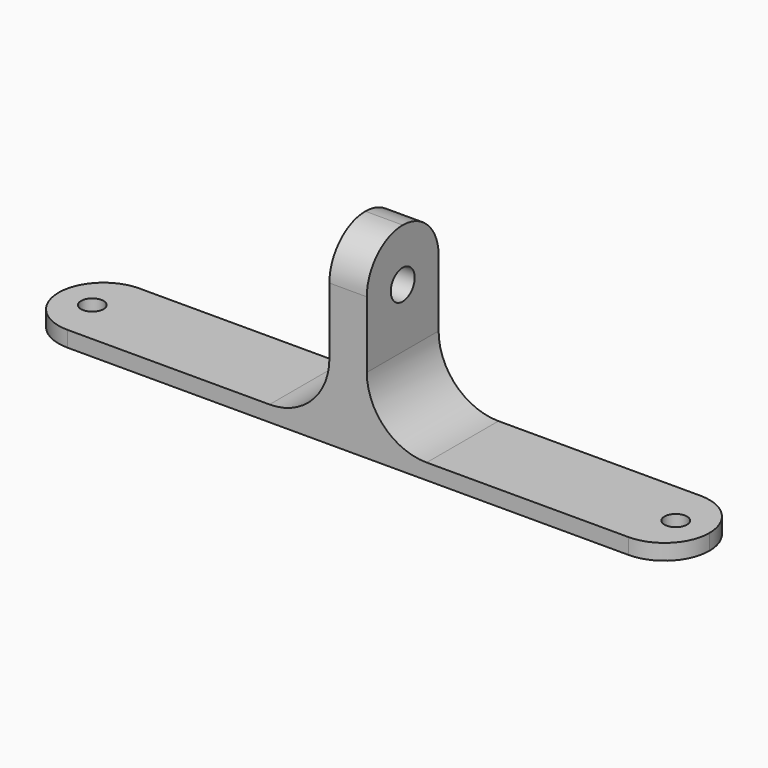
from build123d import *

# Parameters (mm, degrees)
F0_W     = 41
F0_H     = 12
F0_R     = 1.5
F0_W_2   = 5
F1_DEPTH = 2.1
F2_DEPTH = 25
F3_R     = 2
F4_DEPTH = 12.5
F5_R     = 5.99999
F6_R     = 8


# Not quite as in the source:
# - a fillet or chamfer is up to 0.001 mm smaller than in the source, because OpenCascade refuses the exact size


with BuildPart() as f1:
    # F0 (on Top) → F1 (new body)
    with BuildSketch(Plane.XY):
        with Locations((-23, 0)):
            Rectangle(F0_W, F0_H)
        with Locations((-39, 0)):
            Circle(F0_R, mode=Mode.SUBTRACT)
        Rectangle(F0_W_2, F0_H)
        with Locations((23, 0)):
            Rectangle(F0_W, F0_H)
        with Locations((39, 0)):
            Circle(F0_R, mode=Mode.SUBTRACT)
    extrude(amount=F1_DEPTH)

    # F0 (on Top) → F2 (join)
    with BuildSketch(Plane.XY):
        Rectangle(F0_W_2, F0_H)
    extrude(amount=F2_DEPTH)

    # F3 (on Right) → F4 (cut, symmetric)
    with BuildSketch(Plane.YZ):
        with Locations((0, 18)):
            Circle(F3_R)
    extrude(amount=F4_DEPTH, both=True, mode=Mode.SUBTRACT)

    # F5 (radius 6 in the source; OpenCascade refuses exactly that, so slightly less here)
    f5_edges = [f1.edges().sort_by_distance(p)[0] for p in [
        (0, -6, 25),
        (0, 6, 25),
        (-43.5, -6, 1.05),
        (-43.5, 6, 1.05),
        (43.5, -6, 1.05),
        (43.5, 6, 1.05),
    ]]
    fillet(f5_edges, radius=F5_R)

    # F6
    f6_edges = [f1.edges().sort_by_distance(p)[0] for p in [
        (2.5, 0, 2.1),
        (-2.5, 0, 2.1),
    ]]
    fillet(f6_edges, radius=F6_R)


solid = f1.part
